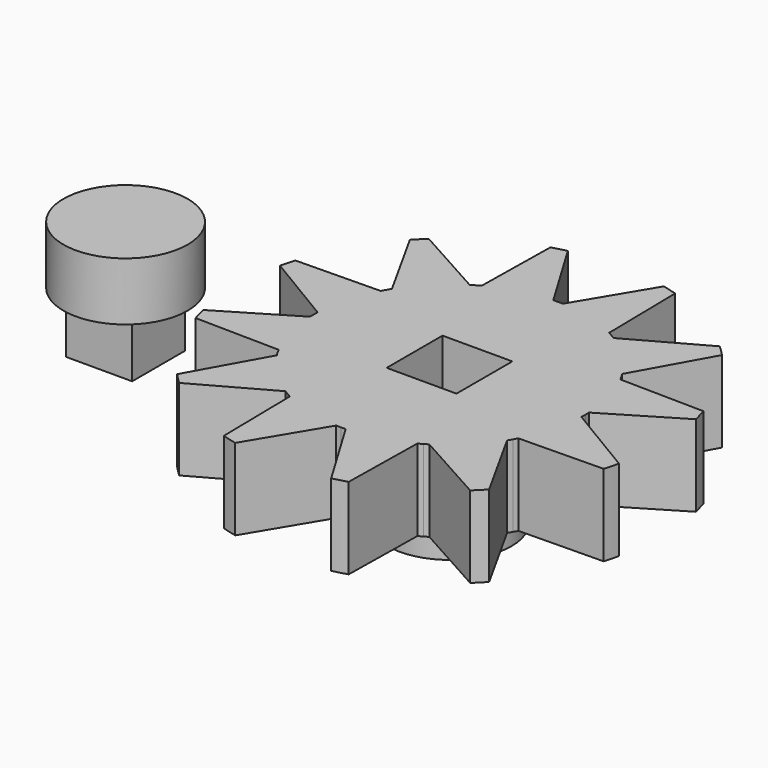
from build123d import *

# Parameters (mm, degrees)
F0_R            = 11
F1_DEPTH        = 4.2
F3_DEPTH        = 4.201
F3_COPIES_COUNT = 12
F5_R            = 3.2
F6_DEPTH        = 3
F7_W            = 3.6
F7_H            = 3.6
F8_DEPTH        = 7.201
F9_R            = 3.2
F10_DEPTH       = 3
F11_W           = 3.4
F11_H           = 3.4
F12_DEPTH       = 3


# Not quite as in the source:
# - a pattern or mirror of a feature is missing from the dataset's text; its kind, count and spacing are read off the source's solid


with BuildPart() as f1:
    # F0 (on Top) → F1 (new body)
    with BuildSketch(Plane.XY):
        Circle(F0_R)
    extrude(amount=F1_DEPTH)

    # F2 (on face) → F3 (cut, through all)
    with BuildSketch(Plane(origin=(0, 0, 0), x_dir=(1, 0, 0), z_dir=(0, 0, -1))):
        with BuildLine():
            ThreePointArc((-6.9957357891, -0.2442964769), (-6.9989338661, -0.1221668451), (-7, 0))
            Line((-7, 0), (-11, 0))
            ThreePointArc((-11, 0), (-10.9292904124, -1.2452353514), (-10.7180707126, -2.4744615978))
            Line((-10.7180707126, -2.4744615978), (-6.9957357891, -0.2442964769))
        make_face()
        with BuildLine():
            Line((-11, 0), (-7, 0))
            ThreePointArc((-7, 0), (-6.9989338661, 0.1221668451), (-6.9957357891, 0.2442964769))
            Line((-6.9957357891, 0.2442964769), (-10.7180707126, 2.4744615978))
            ThreePointArc((-10.7180707126, 2.4744615978), (-10.9292904124, 1.2452353514), (-11, 0))
        make_face()
    f3 = extrude(amount=-F3_DEPTH, mode=Mode.SUBTRACT)

    # F3_copies: F3 ×12 about axis
    f3_copies_axis = Axis((0, 0, 0), (0, 0, 1))
    for i in range(1, F3_COPIES_COUNT):
        add(f3.rotate(f3_copies_axis, i * 360 / F3_COPIES_COUNT), mode=Mode.SUBTRACT)

    # F5 (on face) → F6 (join)
    with BuildSketch(Plane(origin=(0, 0, 0), x_dir=(1, 0, 0), z_dir=(0, 0, -1))):
        Circle(F5_R)
    extrude(amount=F6_DEPTH)

    # F7 (on face) → F8 (cut, through all)
    with BuildSketch(Plane(origin=(0, 0, -3), x_dir=(1, 0, 0), z_dir=(0, 0, -1))):
        Rectangle(F7_W, F7_H)
    extrude(amount=-F8_DEPTH, mode=Mode.SUBTRACT)


with BuildPart() as f10:
    # F9 (on Top) → F10 (new body)
    with BuildSketch(Plane.XY):
        with Locations((-23.0069868267, 7.8802704811)):
            Circle(F9_R)
    extrude(amount=-F10_DEPTH)

    # F11 (on face) → F12 (join)
    with BuildSketch(Plane(origin=(0, 0, -3), x_dir=(1, 0, 0), z_dir=(0, 0, -1))):
        with Locations((-23.0069868267, -7.8802704811)):
            Rectangle(F11_W, F11_H)
    extrude(amount=F12_DEPTH)


solid = Compound([f1.part, f10.part])
